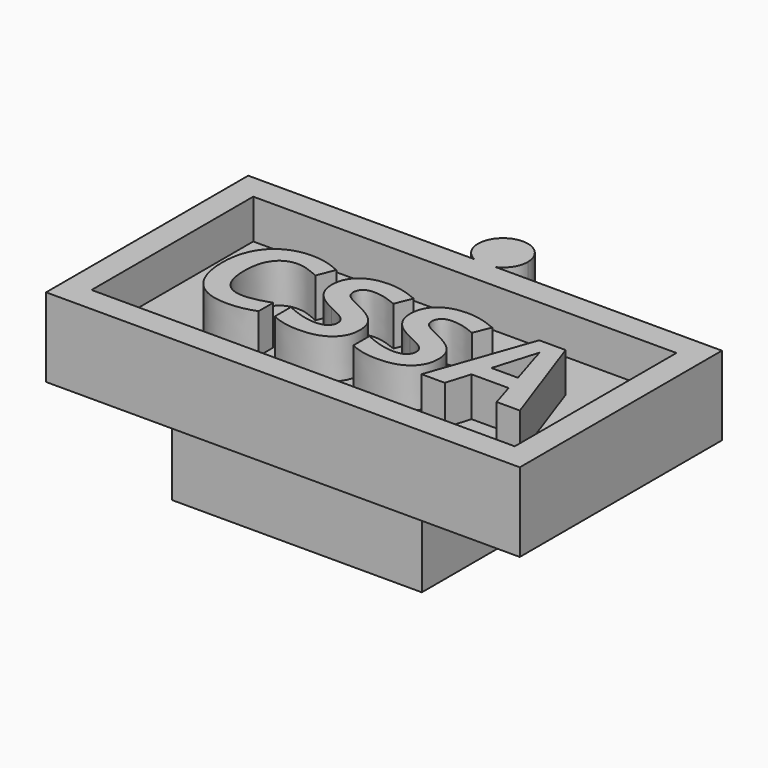
from build123d import *

# Parameters (mm, degrees)
F1_DEPTH     = 3.175
F2_W         = 17.018
F2_H         = 8.128
F3_DEPTH     = 1.5875
F4_W         = 10.05
F4_H         = 8.76
F5_DEPTH     = 3
F6_R         = 3.5
F7_DEPTH     = 3.5
F8_TEXT_SIZE = 5.7333333333
F9_DEPTH     = 1.5875


# Not quite as in the source:
# - Text() gives the source's letters only with a copy of the font that has no kerning and outlines rounded to 1/6400 em; it was checked with that copy


with BuildPart() as f1:
    # F0 (on Top) → F1 (new body)
    with BuildSketch(Plane.XY):
        with BuildLine():
            Line((-9.9608898944, 10.16), (-19.05, 10.16))
            Line((-19.05, 10.16), (-19.05, 0))
            Line((-19.05, 0), (0, 0))
            Line((0, 0), (0, 10.16))
            Line((0, 10.16), (-9.0891101056, 10.16))
            ThreePointArc((-9.0891101056, 10.16), (-9.525, 10.06), (-9.9608898944, 10.16))
        make_face()
        with BuildLine():
            ThreePointArc((-8.525, 11.06), (-10.0560885546, 11.9073163206), (-9.9608898944, 10.16))
            Line((-9.9608898944, 10.16), (-9.0891101056, 10.16))
            ThreePointArc((-9.0891101056, 10.16), (-8.6776836794, 10.5289114454), (-8.525, 11.06))
        make_face()
        with BuildLine():
            Line((-9.0891101056, 10.16), (-9.9608898944, 10.16))
            ThreePointArc((-9.9608898944, 10.16), (-9.525, 10.06), (-9.0891101056, 10.16))
        make_face()
    extrude(amount=F1_DEPTH)

    # F2 (on face) → F3 (cut)
    with BuildSketch(Plane.XY.offset(3.175)):
        with Locations((-9.525, 5.08)):
            Rectangle(F2_W, F2_H)
    extrude(amount=-F3_DEPTH, mode=Mode.SUBTRACT)

    # F4 (on face) → F5 (join)
    with BuildSketch(Plane(origin=(0, 0, 0), x_dir=(1, 0, 0), z_dir=(0, 0, -1))):
        with Locations((-9.525, -5.08)):
            Rectangle(F4_W, F4_H)
    extrude(amount=F5_DEPTH)

    # F6 (on face) → F7 (cut)
    with BuildSketch(Plane(origin=(0, 0, -3), x_dir=(1, 0, 0), z_dir=(0, 0, -1))):
        with Locations((-9.525, -5.08)):
            Circle(F6_R)
    extrude(amount=-F7_DEPTH, mode=Mode.SUBTRACT)

    # F8 (on face) → F9 (join, through all)
    with BuildSketch(Plane.XY.offset(1.5875)):
        with Locations((-16.334, 3.016)):
            Text('CSSA', F8_TEXT_SIZE, font='Open Sans', font_style=FontStyle.BOLD, text_align=(TextAlign.LEFT, TextAlign.BOTTOM))
    extrude(amount=F9_DEPTH)


solid = f1.part
